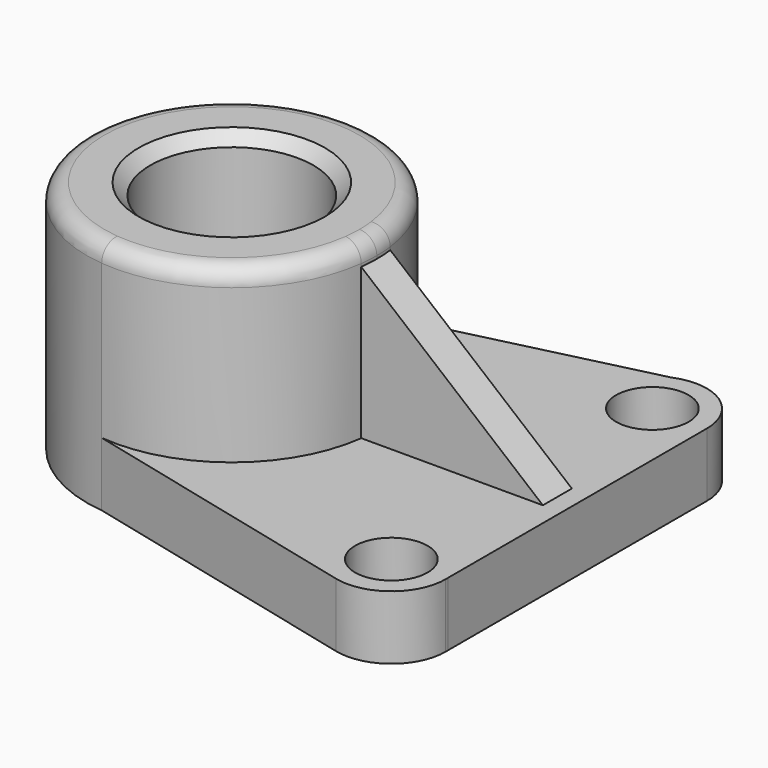
from build123d import *

# Parameters (mm, degrees)
F0_R     = 14.2875
F1_DEPTH = 41.148
F0_R_2   = 6.35
F2_DEPTH = 11.176
F3_DEPTH = 37.592
F5_DEPTH = 127
F6_DEPTH = 76.2
F7_R     = 3.048
F8_SIZE2 = 2.032
F8_SIZE  = 2.032
F9_SIZE2 = 2.032
F9_SIZE  = 2.032


# Not quite as in the source:
# - ends of sketch curves that miss each other by under 0.0002 mm in the source are joined


with BuildPart() as f1:
    # F0 (on Top) → F1 (new body)
    with BuildSketch(Plane.XY):
        with BuildLine():
            ThreePointArc((-17.226482478, 3.175), (-26.6125443992, 19.8759818106), (-44.9953409853, 25.2698432749))
            ThreePointArc((-44.9953409853, 25.2698432749), (-67.8272637159, 0), (-44.9953409853, -25.2698432749))
            ThreePointArc((-44.9953409853, -25.2698432749), (-26.6125443992, -19.8759818106), (-17.226482478, -3.175))
            Line((-17.226482478, -3.175), (-23.8334226287, -3.175))
            Line((-23.8334226287, -3.175), (-23.8334226287, 3.175))
            Line((-23.8334226287, 3.175), (-17.226482478, 3.175))
        make_face()
        with Locations((-42.4272637159, 0)):
            Circle(F0_R, mode=Mode.SUBTRACT)
        with BuildLine():
            ThreePointArc((-17.0272637159, 0), (-17.0771173313, 1.5906219786), (-17.226482478, 3.175))
            Line((-17.226482478, 3.175), (-23.8334226287, 3.175))
            Line((-23.8334226287, 3.175), (-23.8334226287, -3.175))
            Line((-23.8334226287, -3.175), (-17.226482478, -3.175))
            ThreePointArc((-17.226482478, -3.175), (-17.0771173313, -1.5906219786), (-17.0272637159, 0))
        make_face()
    extrude(amount=F1_DEPTH)

    # F0 (on Top) → F2 (join)
    with BuildSketch(Plane.XY):
        with BuildLine():
            Line((4.6864668266, 37.3577696364), (-44.9953409853, 25.2698432749))
            ThreePointArc((-44.9953409853, 25.2698432749), (-26.6125443992, 19.8759818106), (-17.226482478, 3.175))
            Line((-17.226482478, 3.175), (14.5881694606, 3.175))
            Line((14.5881694606, 3.175), (14.5881694606, -3.175))
            Line((14.5881694606, -3.175), (-17.226482478, -3.175))
            ThreePointArc((-17.226482478, -3.175), (-26.6125443992, -19.8759818106), (-44.9953409853, -25.2698432749))
            Line((-44.9953409853, -25.2698432749), (6.0998825197, -37.8248519321))
            ThreePointArc((6.0998825197, -37.8248519321), (2.2878291463, -21.247003676), (17.8827435435, -28.0407838216))
            Line((17.8827435435, -28.0407838216), (17.8977366181, 28.575))
            ThreePointArc((17.8977366181, 28.575), (3.0995063243, 20.6428709799), (4.6864668266, 37.3577696364))
        make_face()
        with BuildLine():
            ThreePointArc((17.8827435435, -28.0407838216), (2.2878291463, -21.247003676), (6.0998825197, -37.8248519321))
            ThreePointArc((6.0998825197, -37.8248519321), (14.2496697061, -36.0708174039), (17.8977362841, -28.575))
            ThreePointArc((17.8977362841, -28.575), (17.8939873612, -28.307786739), (17.8827435435, -28.0407838216))
        make_face()
        with Locations((8.3727362841, -28.575)):
            Circle(F0_R_2, mode=Mode.SUBTRACT)
        with BuildLine():
            ThreePointArc((4.6864668266, 37.3577696364), (3.0995063243, 20.6428709799), (17.8977362841, 28.575))
            ThreePointArc((17.8977362841, 28.575), (13.6459662439, 36.5071290201), (4.6864668266, 37.3577696364))
        make_face()
        with Locations((8.3727362841, 28.575)):
            Circle(F0_R_2, mode=Mode.SUBTRACT)
        with BuildLine():
            Line((14.5881694606, 3.175), (-17.226482478, 3.175))
            ThreePointArc((-17.226482478, 3.175), (-17.0771173313, 1.5906219786), (-17.0272637159, 0))
            ThreePointArc((-17.0272637159, 0), (-17.0771173313, -1.5906219786), (-17.226482478, -3.175))
            Line((-17.226482478, -3.175), (14.5881694606, -3.175))
            Line((14.5881694606, -3.175), (14.5881694606, 3.175))
        make_face()
        with Locations((8.3727362841, 28.575)):
            Circle(F0_R_2)
        with Locations((8.3727362841, -28.575)):
            Circle(F0_R_2)
        with BuildLine():
            ThreePointArc((-17.0272637159, 0), (-17.0771173313, 1.5906219786), (-17.226482478, 3.175))
            Line((-17.226482478, 3.175), (-23.8334226287, 3.175))
            Line((-23.8334226287, 3.175), (-23.8334226287, -3.175))
            Line((-23.8334226287, -3.175), (-17.226482478, -3.175))
            ThreePointArc((-17.226482478, -3.175), (-17.0771173313, -1.5906219786), (-17.0272637159, 0))
        make_face()
    extrude(amount=F2_DEPTH)

    # F0 (on Top) → F3 (join)
    with BuildSketch(Plane.XY):
        with BuildLine():
            Line((14.5881694606, 3.175), (-17.226482478, 3.175))
            ThreePointArc((-17.226482478, 3.175), (-17.0771173313, 1.5906219786), (-17.0272637159, 0))
            ThreePointArc((-17.0272637159, 0), (-17.0771173313, -1.5906219786), (-17.226482478, -3.175))
            Line((-17.226482478, -3.175), (14.5881694606, -3.175))
            Line((14.5881694606, -3.175), (14.5881694606, 3.175))
        make_face()
    extrude(amount=F3_DEPTH)

    # F4 (on face) → F5 (cut)
    with BuildSketch(Plane.XZ.offset(3.175)):
        Polygon((14.5881694606, 37.592), (-17.226482478, 37.592), (14.5881694606, 11.176), align=None)
    extrude(amount=-F5_DEPTH, mode=Mode.SUBTRACT)

    # F0 (on Top) → F6 (cut)
    with BuildSketch(Plane.XY):
        with Locations((8.3727362841, 28.575)):
            Circle(F0_R_2)
        with Locations((8.3727362841, -28.575)):
            Circle(F0_R_2)
    extrude(amount=F6_DEPTH, mode=Mode.SUBTRACT)

    # F7
    f7_edges = [f1.edges().sort_by_distance(p)[0] for p in [
        (-39.859186, -25.269843, 41.148),
    ]]
    fillet(f7_edges, radius=F7_R)

    # F8
    f8_edges = [f1.edges().sort_by_distance(p)[0] for p in [
        (-56.714764, 0, 41.148),
        (-40.167356, -22.237462, 41.148),
    ]]
    chamfer(f8_edges, length=F8_SIZE, length2=F8_SIZE2)

    # F9
    f9_edges = [f1.edges().sort_by_distance(p)[0] for p in [
        (-56.714764, 0, 0),
    ]]
    chamfer(f9_edges, length=F9_SIZE, length2=F9_SIZE2)


solid = f1.part
